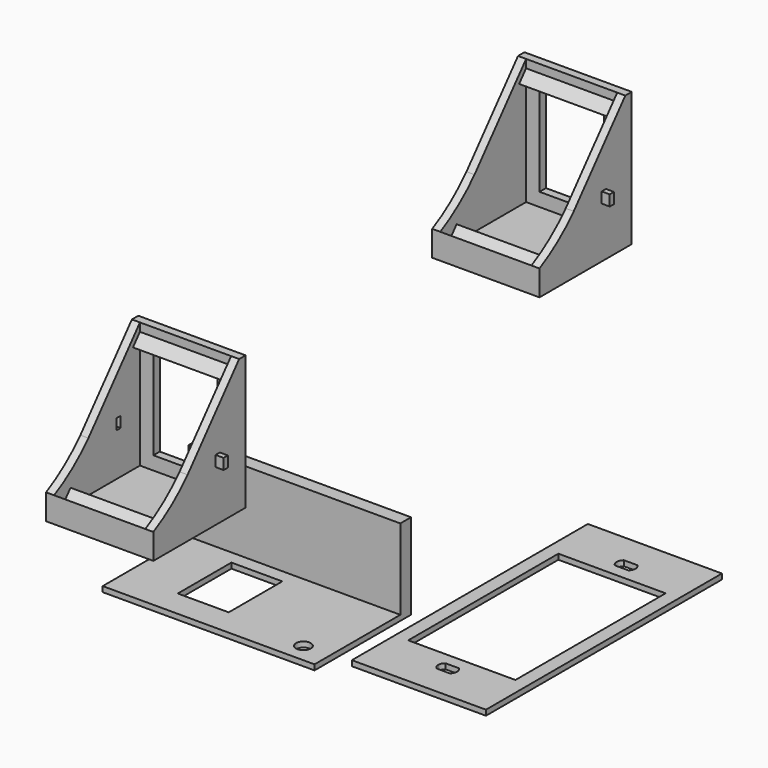
from build123d import *

# Parameters (mm, degrees)
F0_W           = 40
F0_H           = 50
F0_W_2         = 24
F0_H_2         = 38
F1_DEPTH       = 3
F2_W           = 40
F2_H           = 3
F3_DEPTH       = 40
F5_DEPTH       = 3
F7_DEPTH       = 3
F8_W           = 3
F8_H           = 2.8935517733
F9_DEPTH       = 34
F11_DEPTH      = 37
F11_DEPTH_BACK = 3
F13_DEPTH      = 34
F14_W          = 2
F14_H          = 4
F15_DEPTH      = 3
F16_W          = 2
F16_H          = 4
F17_DEPTH      = 25
F19_DEPTH      = 3
F21_DEPTH      = 3
F23_W          = 2
F23_H          = 4
F24_DEPTH      = 3
F25_W          = 50
F25_H          = 110
F26_DEPTH      = 2
F28_DEPTH      = 25
F29_W          = 5
F29_H          = 4.2
F30_DEPTH      = 25
F32_W          = 79
F32_H          = 45
F32_W_2        = 19
F32_H_2        = 25
F33_DEPTH      = 2
F34_W          = 79
F34_H          = 5
F35_DEPTH      = 30
F36_R          = 2.75
F37_DEPTH      = 25


with BuildPart() as f1:
    # F0 (on Front) → F1 (new body)
    with BuildSketch(Plane.XZ):
        with Locations((-40, 45)):
            Rectangle(F0_W, F0_H)
        with Locations((-40, 47)):
            Rectangle(F0_W_2, F0_H_2, mode=Mode.SUBTRACT)
    extrude(amount=F1_DEPTH)

    # F2 (on face) → F3 (join)
    with BuildSketch(Plane.XZ.offset(3)):
        with Locations((-40, 21.5)):
            Rectangle(F2_W, F2_H)
    extrude(amount=F3_DEPTH)

    # F4 (on face) → F5 (join)
    with BuildSketch(Plane(origin=(-60, 0, 0), x_dir=(0, -1, 0), z_dir=(-1, 0, 0))):
        Polygon((43, 23), (3, 70), (3, 23), align=None)
    extrude(amount=-F5_DEPTH)

    # F6 (on face) → F7 (join)
    with BuildSketch(Plane.YZ.offset(-20)):
        Polygon((-3, 70), (-43, 23), (-3, 23), align=None)
    extrude(amount=-F7_DEPTH)

    # F8 (on face) → F9 (join, through all)
    with BuildSketch(Plane.YZ.offset(-57)):
        Polygon((-3, 66), (-3, 66.9141451752), (-6.2405931476, 63.1064482267), (-3, 63.1064482267), align=None)
        with Locations((-1.5, 64.5532241133)):
            Rectangle(F8_W, F8_H)
    extrude(amount=F9_DEPTH)

    # F10 (on face) → F11 (join, two sides)
    with BuildSketch(Plane.YZ.offset(-57)) as f11_sk:
        Polygon((-43, 23), (-35.3625, 23), (-43, 29.5), align=None)
    extrude(amount=F11_DEPTH)
    extrude(f11_sk.sketch, amount=-F11_DEPTH_BACK)

    # F12 (on face) → F13 (join, through all)
    with BuildSketch(Plane.YZ.offset(-57)):
        Polygon((-35.3625, 28.8882076752), (-38.2687300943, 25.4733873143), (-35.3625, 23), align=None)
    extrude(amount=F13_DEPTH)

    # F14 (on face) → F15 (join)
    with BuildSketch(Plane.YZ.offset(-20)):
        with Locations((-13, 41)):
            Rectangle(F14_W, F14_H)
    extrude(amount=F15_DEPTH)

    # F16 (on face) → F17 (cut)
    with BuildSketch(Plane(origin=(-60, 0, 0), x_dir=(0, -1, 0), z_dir=(-1, 0, 0))):
        with Locations((13, 41)):
            Rectangle(F16_W, F16_H)
    extrude(amount=-F17_DEPTH, mode=Mode.SUBTRACT)

    # F18 (on face) → F19 (join, through all)
    with BuildSketch(Plane(origin=(-60, 0, 0), x_dir=(0, -1, 0), z_dir=(-1, 0, 0))):
        with BuildLine():
            ThreePointArc((43, 29.5), (34.4666549031, 34.9236078783), (27.0258514269, 41.7696245734))
            Line((27.0258514269, 41.7696245734), (39.7918088737, 26.7696245734))
            Line((39.7918088737, 26.7696245734), (43, 29.5))
        make_face()
    extrude(amount=-F19_DEPTH)

    # F20 (on face) → F21 (join, through all)
    with BuildSketch(Plane.YZ.offset(-20)):
        with BuildLine():
            ThreePointArc((-27.0258514269, 41.7696245734), (-34.4666549031, 34.9236078783), (-43, 29.5))
            Line((-43, 29.5), (-39.7918088737, 26.7696245734))
            Line((-39.7918088737, 26.7696245734), (-27.0258514269, 41.7696245734))
        make_face()
    extrude(amount=-F21_DEPTH)


with BuildPart() as f22_1:
    # F22: copy of F1
    add(f1.part.moved(Location((80, 80, 80))))

    # F23 (on face) → F24 (join, through all)
    with BuildSketch(Plane(origin=(20, 0, 0), x_dir=(0, -1, 0), z_dir=(-1, 0, 0))):
        with Locations((-67, 121)):
            Rectangle(F23_W, F23_H)
    extrude(amount=-F24_DEPTH)


with BuildPart() as f26:
    # F25 (on Top) → F26 (new body)
    with BuildSketch(Plane.XY):
        with Locations((67.6461342699, 26.2317729229)):
            Rectangle(F25_W, F25_H)
    extrude(amount=F26_DEPTH)

    # F27 (on face) → F28 (cut)
    with BuildSketch(Plane(origin=(0, 0, 0), x_dir=(1, 0, 0), z_dir=(0, 0, -1))):
        Polygon((63.6029914021, -61.2317729229), (87.6461342699, -61.2317729229), (87.6461342699, -35.5290547013), (87.6461342699, 8.7682270771), (62.8203749657, 8.7682270771), (47.6461342699, 8.7682270771), (47.6461342699, -35.5290547013), (47.6461342699, -61.2317729229), align=None)
    extrude(amount=-F28_DEPTH, mode=Mode.SUBTRACT)

    # F29 (on face) → F30 (cut)
    with BuildSketch(Plane(origin=(0, 0, 0), x_dir=(1, 0, 0), z_dir=(0, 0, -1))):
        with BuildLine():
            ThreePointArc((71.1461342699, 15.3682270771), (70.8833719733, 16.5311974121), (70.1461342699, 17.4682270771))
            Line((70.1461342699, 17.4682270771), (70.1461342699, 13.2682270771))
            ThreePointArc((70.1461342699, 13.2682270771), (70.8833719733, 14.2052567421), (71.1461342699, 15.3682270771))
        make_face()
        with Locations((67.6461342699, 15.3682270771)):
            Rectangle(F29_W, F29_H)
        with BuildLine():
            Line((65.1461342699, 13.2682270771), (65.1461342699, 17.4682270771))
            ThreePointArc((65.1461342699, 17.4682270771), (64.4088965616, 16.5311974019), (64.1461342699, 15.3682270546))
            ThreePointArc((64.1461342699, 15.3682270546), (64.4088965713, 14.205256732), (65.1461342699, 13.2682270771))
        make_face()
        with Locations((67.6461342699, -67.8317729229)):
            Rectangle(F29_W, F29_H)
        with BuildLine():
            Line((70.1461342699, -65.7317729229), (70.1461342699, -69.9317729229))
            ThreePointArc((70.1461342699, -69.9317729229), (70.8833719733, -68.9947432579), (71.1461342699, -67.8317729229))
            ThreePointArc((71.1461342699, -67.8317729229), (70.8833719733, -66.6688025879), (70.1461342699, -65.7317729229))
        make_face()
        with BuildLine():
            ThreePointArc((64.1461342699, -67.8317729229), (64.4088965665, -68.9947432579), (65.1461342699, -69.9317729229))
            Line((65.1461342699, -69.9317729229), (65.1461342699, -65.7317729229))
            ThreePointArc((65.1461342699, -65.7317729229), (64.4088965665, -66.6688025879), (64.1461342699, -67.8317729229))
        make_face()
    extrude(amount=-F30_DEPTH, mode=Mode.SUBTRACT)


with BuildPart() as f33:
    # F32 (on face) → F33 (new body)
    with BuildSketch(Plane.XY):
        with Locations((-3.6956531787, -15.1206750181)):
            Rectangle(F32_W, F32_H)
        with Locations((-13.6956531787, -15.1206750181)):
            Rectangle(F32_W_2, F32_H_2, mode=Mode.SUBTRACT)
    extrude(amount=F33_DEPTH)

    # F34 (on face) → F35 (join)
    with BuildSketch(Plane.XY.offset(2)):
        with Locations((-3.6956531787, 4.8793249819)):
            Rectangle(F34_W, F34_H)
    extrude(amount=F35_DEPTH)

    # F36 (on face) → F37 (cut)
    with BuildSketch(Plane(origin=(0, 0, 0), x_dir=(1, 0, 0), z_dir=(0, 0, -1))):
        with Locations((25.9792152792, 30.5160041898)):
            Circle(F36_R)
    extrude(amount=-F37_DEPTH, mode=Mode.SUBTRACT)


solid = Compound([f1.part, f22_1.part, f26.part, f33.part])
